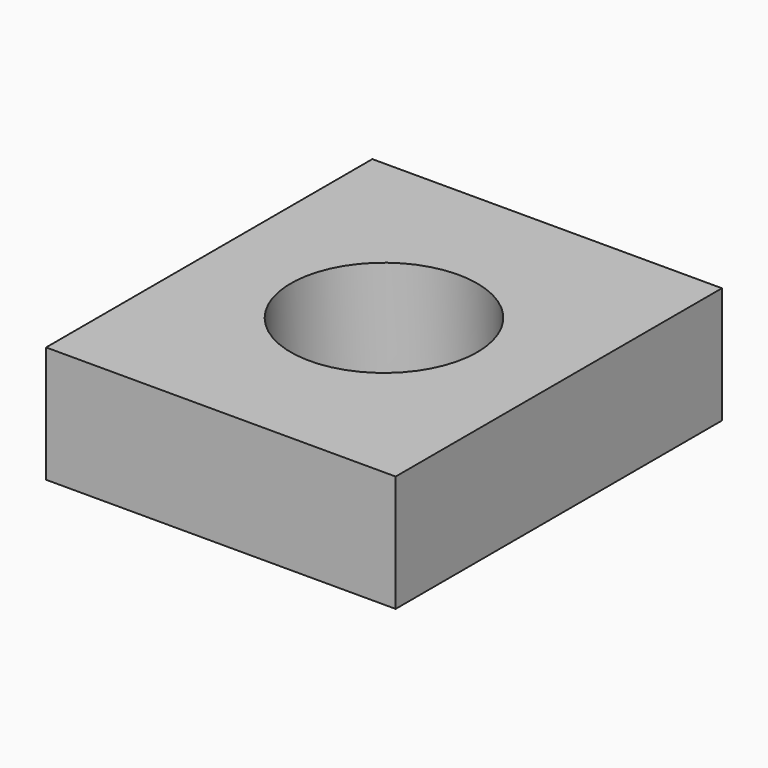
from build123d import *

# Parameters (mm, degrees)
F0_W     = 6
F0_H     = 7
F0_R     = 1.6
F1_DEPTH = 4
F2_DEPTH = 2


# Not quite as in the source:
# - a feature names something its author has since deleted; it is built from what else it names


with BuildPart() as f1:
    # F0 (on Top) → F1 (new body)
    with BuildSketch(Plane.XY):
        Rectangle(F0_W, F0_H)
        Circle(F0_R, mode=Mode.SUBTRACT)
    extrude(amount=-F1_DEPTH)

    # F0 (on Top) → F2 (cut)
    with BuildSketch(Plane.XY):
        Rectangle(F0_W, F0_H)
        Circle(F0_R, mode=Mode.SUBTRACT)
    extrude(amount=-F2_DEPTH, mode=Mode.SUBTRACT)


solid = f1.part
